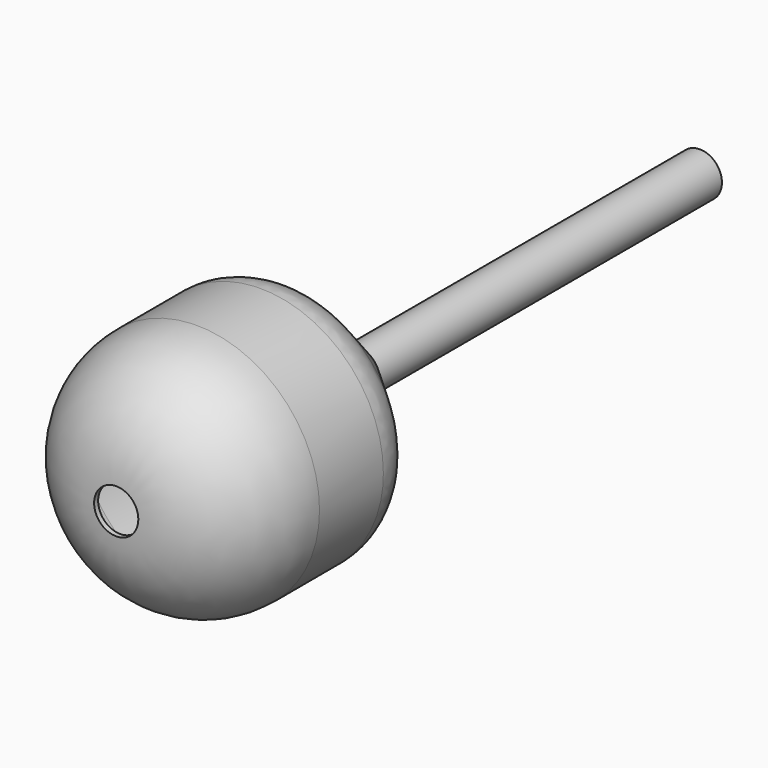
from build123d import *

# Parameters (mm, degrees)
F0_R     = 61.9549494039
F1_DEPTH = 25.4
F2_DEPTH = 127
F3_R     = 50.8
F4_SIZE  = 50.8
F5_T     = -2.54
F6_R     = 11.1549494039
F9_R     = 25.4


# Not quite as in the source:
# - a shell that OpenCascade refuses in one call is made with other operations: the cavity is built on its own and cut out


with BuildPart() as f1:
    # F0 (on Front) → F1 (new body)
    with BuildSketch(Plane.XZ):
        Circle(F0_R)
    extrude(amount=F1_DEPTH)

    # F2 (add): a face of the model
    f2_faces = [f1.faces().sort_by_distance(p)[0] for p in [
        (0, -25.4, 0),
    ]]
    extrude(f2_faces, amount=F2_DEPTH)

    # F3
    f3_edges = [f1.edges().sort_by_distance(p)[0] for p in [
        (-61.954949, -152.4, 0),
    ]]
    fillet(f3_edges, radius=F3_R)

    # F4
    f4_edges = [f1.edges().sort_by_distance(p)[0] for p in [
        (-61.954949, 0, 0),
    ]]
    chamfer(f4_edges, length=F4_SIZE)

    # F5: a shell. OpenCascade refuses it in one call, so the cavity is built on its own and cut out:
    # the body offset inwards by the wall thickness, plus a prism from it out through each open face.
    f5_core = offset(f1.part, amount=F5_T, mode=Mode.PRIVATE)
    f5_exits = [f5_core.faces().sort_by_distance(p)[0] for p in [
        (0, -149.86, 0),
    ]]
    add(f5_core, mode=Mode.SUBTRACT)
    extrude(f5_exits, amount=-F5_T, mode=Mode.SUBTRACT)

    # F8: sweep along a path in F7
    with BuildLine(Plane.YZ) as f8_path:
        Line((215.7490998507, 0), (0, 0))
    # F6 (on face) → F8 (sweep)
    with BuildSketch(Plane(origin=(0, 0, 0), x_dir=(-1, 0, 0), z_dir=(0, 1, 0))):
        Circle(F6_R)
    sweep(path=f8_path.line)

    # F9
    f9_edges = [f1.edges().sort_by_distance(p)[0] for p in [
        (-61.954949, -50.8, 0),
    ]]
    fillet(f9_edges, radius=F9_R)


solid = f1.part
